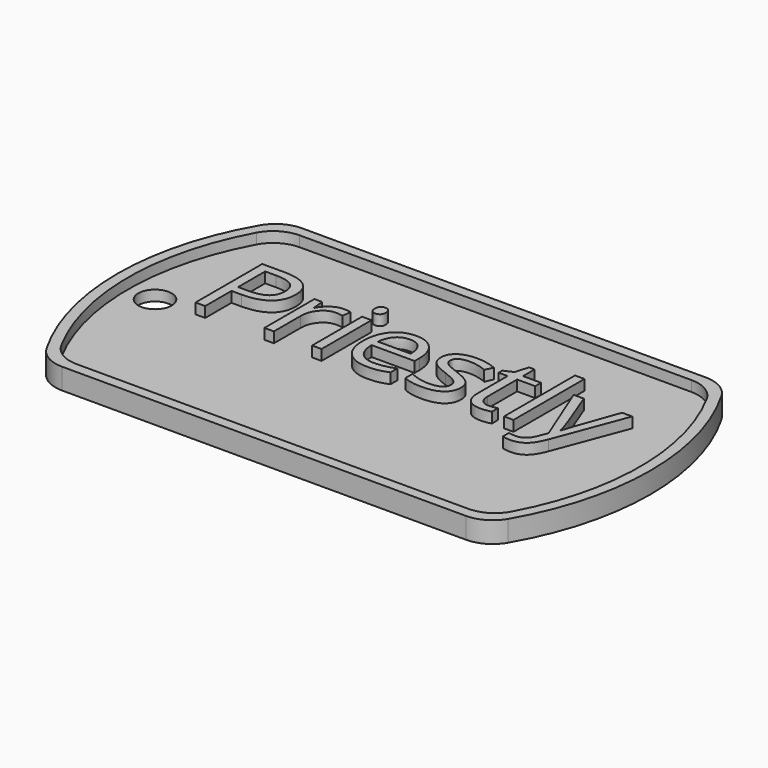
from build123d import *

# Parameters (mm, degrees)
F1_DEPTH     = 1
F3_DEPTH     = 1
F4_R         = 1.5875
F5_DEPTH     = 1
F6_TEXT_SIZE = 11.1260684207
F7_DEPTH     = 1


# Not quite as in the source:
# - Text() gives the source's letters only with a copy of the font that has no kerning and outlines rounded to 1/6400 em; it was checked with that copy


with BuildPart() as f1:
    # F0 (on Top) → F1 (new body)
    with BuildSketch(Plane.XY):
        with BuildLine():
            ThreePointArc((-19.2474145991, 14.2875), (-20.8349145991, 13.862130657), (-21.9970452561, 12.7))
            ThreePointArc((-21.9970452561, 12.7), (-25.4, 0), (-21.9970452561, -12.7))
            ThreePointArc((-21.9970452561, -12.7), (-20.8349145991, -13.862130657), (-19.2474145991, -14.2875))
            Line((-19.2474145991, -14.2875), (19.2474145991, -14.2875))
            ThreePointArc((19.2474145991, -14.2875), (20.8349145991, -13.862130657), (21.9970452561, -12.7))
            ThreePointArc((21.9970452561, -12.7), (25.4, 0), (21.9970452561, 12.7))
            ThreePointArc((21.9970452561, 12.7), (20.8349145991, 13.862130657), (19.2474145991, 14.2875))
            Line((19.2474145991, 14.2875), (-19.2474145991, 14.2875))
        make_face()
    extrude(amount=F1_DEPTH)

    # F2 (on face) → F3 (join)
    with BuildSketch(Plane.XY.offset(1)):
        with BuildLine():
            Line((19.2474145991, 14.2875), (-19.2474145991, 14.2875))
            ThreePointArc((-19.2474145991, 14.2875), (-20.8349145991, 13.862130657), (-21.9970452561, 12.7))
            ThreePointArc((-21.9970452561, 12.7), (-25.4, 0), (-21.9970452561, -12.7))
            ThreePointArc((-21.9970452561, -12.7), (-20.8349145991, -13.862130657), (-19.2474145991, -14.2875))
            Line((-19.2474145991, -14.2875), (19.2474145991, -14.2875))
            ThreePointArc((19.2474145991, -14.2875), (20.8349145991, -13.862130657), (21.9970452561, -12.7))
            ThreePointArc((21.9970452561, -12.7), (25.4, 0), (21.9970452561, 12.7))
            ThreePointArc((21.9970452561, 12.7), (20.8349145991, 13.862130657), (19.2474145991, 14.2875))
        make_face()
        with BuildLine():
            ThreePointArc((-21.4526124879, 11.6252061249), (-20.2856017842, 12.8404540819), (-18.6611352482, 13.2875))
            Line((-18.6611352482, 13.2875), (18.6611352482, 13.2875))
            ThreePointArc((18.6611352482, 13.2875), (20.2856017842, 12.8404540819), (21.4526124879, 11.6252061249))
            ThreePointArc((21.4526124879, 11.6252061249), (24.4, 0), (21.4526124879, -11.6252061249))
            ThreePointArc((21.4526124879, -11.6252061249), (20.2856017842, -12.8404540819), (18.6611352482, -13.2875))
            Line((18.6611352482, -13.2875), (-18.6611352482, -13.2875))
            ThreePointArc((-18.6611352482, -13.2875), (-20.2856017842, -12.8404540819), (-21.4526124879, -11.6252061249))
            ThreePointArc((-21.4526124879, -11.6252061249), (-24.4, 0), (-21.4526124879, 11.6252061249))
        make_face(mode=Mode.SUBTRACT)
    extrude(amount=F3_DEPTH)

    # F4 (on face) → F5 (cut)
    with BuildSketch(Plane.XY.offset(1)):
        with Locations((-21.821282804, 0)):
            Circle(F4_R)
    extrude(amount=-F5_DEPTH, mode=Mode.SUBTRACT)

    # F6 (on face) → F7 (join)
    with BuildSketch(Plane.XY.offset(1)):
        with Locations((-19.0500002354, 0)):
            Text('Priestly', F6_TEXT_SIZE, font='Open Sans', text_align=(TextAlign.LEFT, TextAlign.BOTTOM))
    extrude(amount=F7_DEPTH)


solid = f1.part
